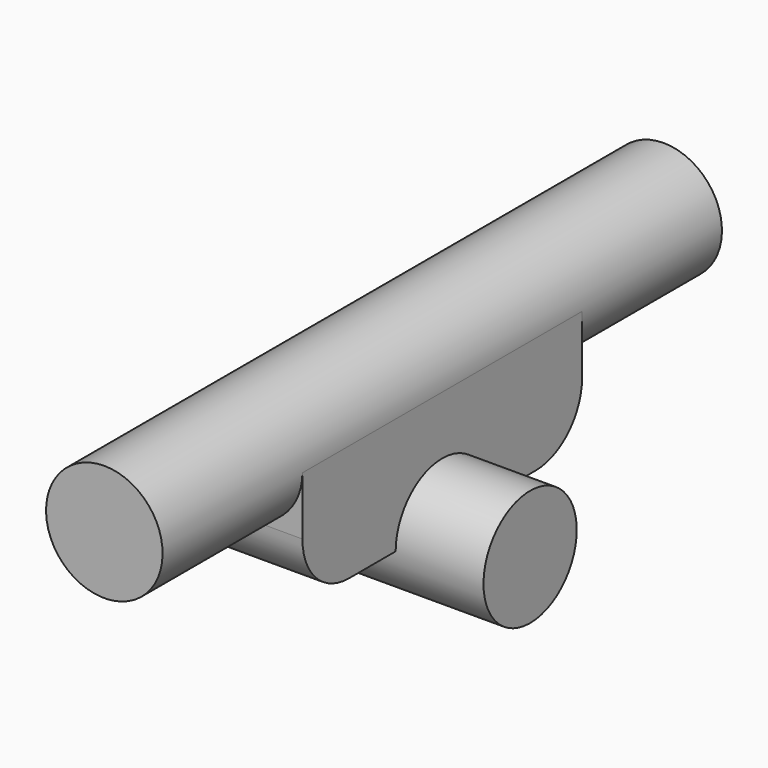
from build123d import *

# Parameters (mm, degrees)
F0_W     = 240
F0_H     = 20
F2_W     = 40
F2_H     = 120
F3_DEPTH = 40
F4_R     = 19.99999
F5_W     = 100
F5_H     = 20


# Not quite as in the source:
# - a fillet or chamfer is up to 0.001 mm smaller than in the source, because OpenCascade refuses the exact size


with BuildPart() as f1:
    # F0 (on Right) → F1 (revolve)
    with BuildSketch(Plane.YZ):
        with Locations((0, 10)):
            Rectangle(F0_W, F0_H)
    revolve(axis=Axis((0, 0, 0), (0, 1, 0)))

    # F2 (on Top) → F3 (join)
    with BuildSketch(Plane.XY):
        Rectangle(F2_W, F2_H)
    extrude(amount=-F3_DEPTH)

    # F4 (radius 20 in the source; OpenCascade refuses exactly that, so slightly less here)
    f4_edges = [f1.edges().sort_by_distance(p)[0] for p in [
        (0, -60, -40),
        (0, 60, -40),
    ]]
    fillet(f4_edges, radius=F4_R)

    # F5 (on Front) → F6 (revolve)
    with BuildSketch(Plane.XZ):
        with Locations((0.1484978533, -50)):
            Rectangle(F5_W, F5_H)
    revolve(axis=Axis((43.9392195031, 0, -40), (1, 0, 0)))


solid = f1.part
